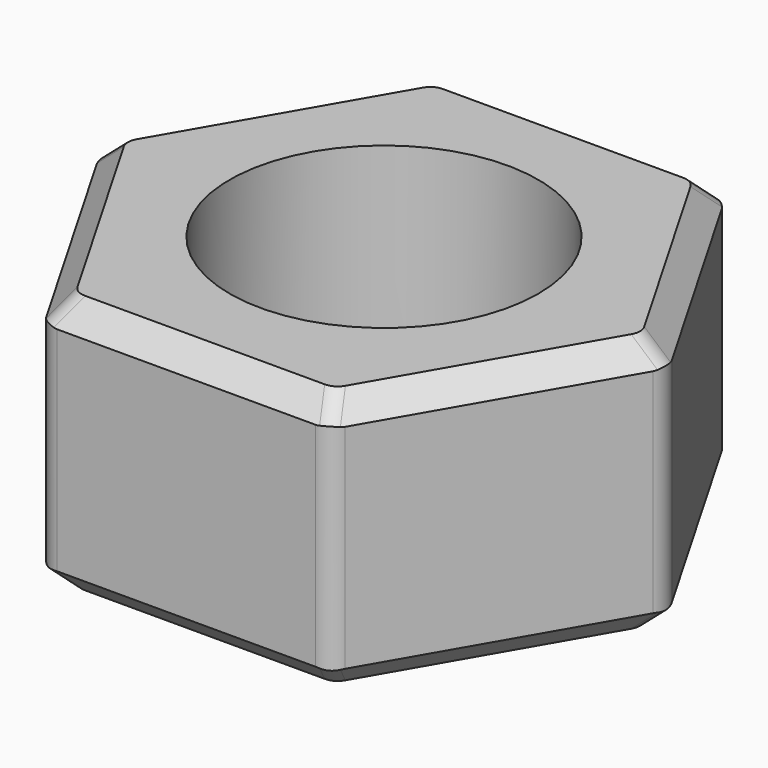
from build123d import *

# Parameters (mm, degrees)
F0_R     = 5
F1_DEPTH = 8.4
F2_SIZE  = 0.75
F3_F1_R  = 0.75
F3_F2_R  = 0.75
F3_F3_R  = 0.75
F3_F4_R  = 0.75
F3_F5_R  = 0.75
F3_F6_R  = 0.75
F3_F7_R  = 0.75
F3_F8_R  = 0.75
F3_F9_R  = 0.75
F3_F10_R = 0.75
F3_F11_R = 0.75
F3_F12_R = 0.75
F3_F13_R = 0.75
F3_F14_R = 0.75
F3_F15_R = 0.75
F3_F16_R = 0.75
F3_F17_R = 0.75
F3_F18_R = 0.75


with BuildPart() as f1:
    # F0 (on Top) → F1 (new body)
    with BuildSketch(Plane.XY):
        Polygon((4.6188021535, 8), (-4.6188021535, 8), (-9.237604307, 0), (-4.6188021535, -8), (4.6188021535, -8), (9.237604307, 0), align=None)
        Circle(F0_R, mode=Mode.SUBTRACT)
    extrude(amount=F1_DEPTH)

    # F2
    f2_edges = [f1.edges().sort_by_distance(p)[0] for p in [
        (0, -8, 8.4),
        (-6.928203, -4, 8.4),
        (-6.928203, 4, 8.4),
        (0, 8, 8.4),
        (6.928203, 4, 8.4),
        (6.928203, -4, 8.4),
        (6.928203, -4, 0),
        (0, -8, 0),
        (-6.928203, -4, 0),
        (-6.928203, 4, 0),
        (0, 8, 0),
        (6.928203, 4, 0),
    ]]
    chamfer(f2_edges, length=F2_SIZE)

    # F3: fillet of radius 0.75 on 18 edges, made by hand

    # F3_f1
    f3_f1_edges = [f1.edges().sort_by_distance(p)[0] for p in [
        (4.6188021535, 8, 4.2),
    ]]
    fillet(f3_f1_edges, radius=F3_F1_R)

    # F3_f2
    f3_f2_edges = [f1.edges().sort_by_distance(p)[0] for p in [
        (-4.6188021535, 8, 4.2),
    ]]
    fillet(f3_f2_edges, radius=F3_F2_R)

    # F3_f3
    f3_f3_edges = [f1.edges().sort_by_distance(p)[0] for p in [
        (9.237604307, 0, 4.2),
    ]]
    fillet(f3_f3_edges, radius=F3_F3_R)

    # F3_f4
    f3_f4_edges = [f1.edges().sort_by_distance(p)[0] for p in [
        (4.3732894516, 7.5747595264, 0.3247595264),
    ]]
    fillet(f3_f4_edges, radius=F3_F4_R)

    # F3_f5
    f3_f5_edges = [f1.edges().sort_by_distance(p)[0] for p in [
        (-4.3732894516, 7.5747595264, 0.3247595264),
    ]]
    fillet(f3_f5_edges, radius=F3_F5_R)

    # F3_f6
    f3_f6_edges = [f1.edges().sort_by_distance(p)[0] for p in [
        (4.3732894516, 7.5747595264, 8.0752404736),
    ]]
    fillet(f3_f6_edges, radius=F3_F6_R)

    # F3_f7
    f3_f7_edges = [f1.edges().sort_by_distance(p)[0] for p in [
        (-4.3732894516, 7.5747595264, 8.0752404736),
    ]]
    fillet(f3_f7_edges, radius=F3_F7_R)

    # F3_f8
    f3_f8_edges = [f1.edges().sort_by_distance(p)[0] for p in [
        (-9.237604307, 0, 4.2),
    ]]
    fillet(f3_f8_edges, radius=F3_F8_R)

    # F3_f9
    f3_f9_edges = [f1.edges().sort_by_distance(p)[0] for p in [
        (4.6188021535, -8, 4.2),
    ]]
    fillet(f3_f9_edges, radius=F3_F9_R)

    # F3_f10
    f3_f10_edges = [f1.edges().sort_by_distance(p)[0] for p in [
        (8.7465789032, 0, 0.3247595264),
    ]]
    fillet(f3_f10_edges, radius=F3_F10_R)

    # F3_f11
    f3_f11_edges = [f1.edges().sort_by_distance(p)[0] for p in [
        (8.7465789032, 0, 8.0752404736),
    ]]
    fillet(f3_f11_edges, radius=F3_F11_R)

    # F3_f12
    f3_f12_edges = [f1.edges().sort_by_distance(p)[0] for p in [
        (-8.7465789032, 0, 0.3247595264),
    ]]
    fillet(f3_f12_edges, radius=F3_F12_R)

    # F3_f13
    f3_f13_edges = [f1.edges().sort_by_distance(p)[0] for p in [
        (-8.7465789032, 0, 8.0752404736),
    ]]
    fillet(f3_f13_edges, radius=F3_F13_R)

    # F3_f14
    f3_f14_edges = [f1.edges().sort_by_distance(p)[0] for p in [
        (-4.6188021535, -8, 4.2),
    ]]
    fillet(f3_f14_edges, radius=F3_F14_R)

    # F3_f15
    f3_f15_edges = [f1.edges().sort_by_distance(p)[0] for p in [
        (4.3732894516, -7.5747595264, 0.3247595264),
    ]]
    fillet(f3_f15_edges, radius=F3_F15_R)

    # F3_f16
    f3_f16_edges = [f1.edges().sort_by_distance(p)[0] for p in [
        (4.3732894516, -7.5747595264, 8.0752404736),
    ]]
    fillet(f3_f16_edges, radius=F3_F16_R)

    # F3_f17
    f3_f17_edges = [f1.edges().sort_by_distance(p)[0] for p in [
        (-4.3732894516, -7.5747595264, 0.3247595264),
    ]]
    fillet(f3_f17_edges, radius=F3_F17_R)

    # F3_f18
    f3_f18_edges = [f1.edges().sort_by_distance(p)[0] for p in [
        (-4.3732894516, -7.5747595264, 8.0752404736),
    ]]
    fillet(f3_f18_edges, radius=F3_F18_R)


solid = f1.part
